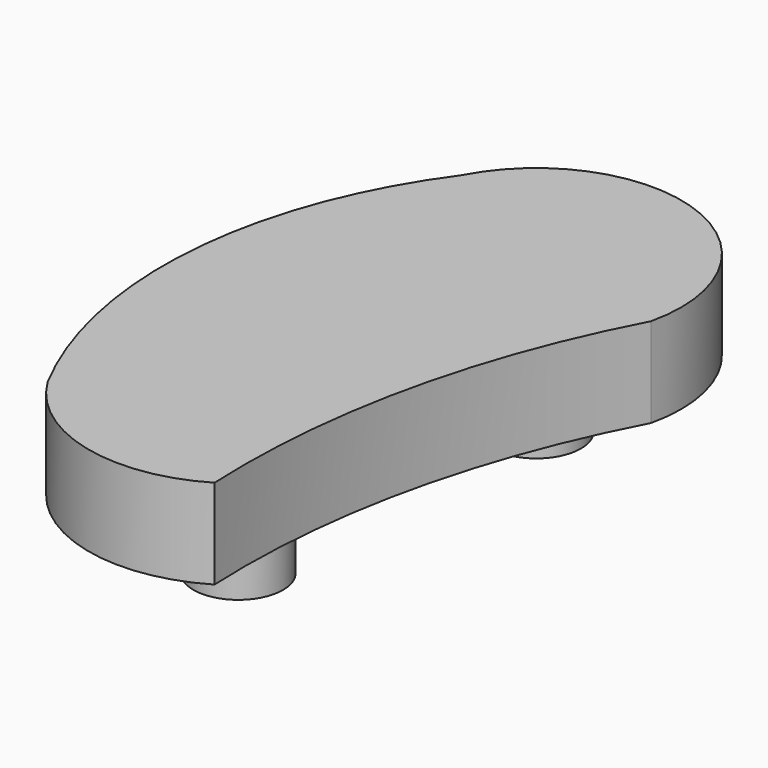
from build123d import *

# Parameters (mm, degrees)
F0_R     = 2
F1_DEPTH = 4
F2_DEPTH = 7


# Not quite as in the source:
# - a feature names something its author has since deleted; it is built from what else it names


with BuildPart() as f1:
    # F0 (on Top) → F1 (new body)
    with BuildSketch(Plane.XY):
        with BuildLine():
            ThreePointArc((8.8045736775, 5.9720319696), (4.7714301194, 13.5077650507), (-3.2184339135, 10.47204557))
            ThreePointArc((-3.2184339135, 10.47204557), (-7.0349525259, 0.086158841), (-4.7456540833, -10.739346695))
            ThreePointArc((-4.7456540833, -10.739346695), (-0.5751322141, -13.8008387314), (4.5426217839, -13.0428280681))
            ThreePointArc((4.5426217839, -13.0428280681), (5.4021565515, -3.2504198201), (8.8045736775, 5.9720319696))
        make_face()
        with Locations((1.0620787063, -7.3684426025)):
            Circle(F0_R, mode=Mode.SUBTRACT)
        with Locations((2.5027735673, 7.4464333818)):
            Circle(F0_R, mode=Mode.SUBTRACT)
    extrude(amount=-F1_DEPTH)

    # F0 (on Top) → F2 (join)
    with BuildSketch(Plane.XY):
        with Locations((2.5027735673, 7.4464333818)):
            Circle(F0_R)
        with Locations((1.0620787063, -7.3684426025)):
            Circle(F0_R)
    extrude(amount=-F2_DEPTH)


solid = f1.part
